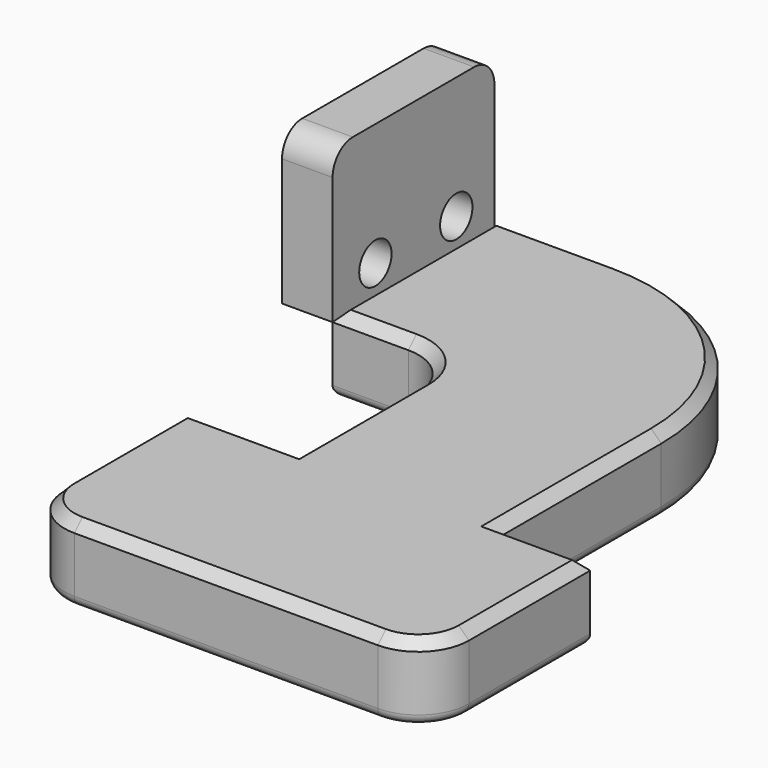
from build123d import *

# Parameters (mm, degrees)
F1_DEPTH = 7.5
F2_DEPTH = 2.5
F3_R     = 1
F4_SIZE  = 1
F5_R     = 2
F6_DEPTH = 5


# Not quite as in the source:
# - a feature names something its author has since deleted; it is built from what else it names


with BuildPart() as f1:
    # F0 (on Top) → F1 (new body)
    with BuildSketch(Plane.XY):
        with BuildLine():
            Line((-15.2574911714, 10), (-27.7574911714, 10))
            Line((-27.7574911714, 10), (-27.7574911714, -10))
            Line((-27.7574911714, -10), (-20.2574911714, -10))
            ThreePointArc((-20.2574911714, -10), (-16.7219572654, -11.4644660941), (-15.2574911714, -15))
            Line((-15.2574911714, -15), (-15.2574911714, -30.0000000031))
            Line((-15.2574911714, -30.0000000031), (4.7425088286, -30.0000000031))
            Line((4.7425088286, -30.0000000031), (4.7425088286, -10))
            ThreePointArc((4.7425088286, -10), (-1.1153555476, 4.1421356237), (-15.2574911714, 10))
        make_face()
        with BuildLine():
            Line((13.7208224833, -30.0000000031), (4.7425088286, -30.0000000031))
            Line((4.7425088286, -30.0000000031), (-15.2574911714, -30.0000000031))
            Line((-15.2574911714, -30.0000000031), (-26.2791775167, -30.0000000031))
            Line((-26.2791775167, -30.0000000031), (-26.2791775167, -45.0000000031))
            ThreePointArc((-26.2791775167, -45.0000000031), (-24.8147114226, -48.535533909), (-21.2791775167, -50.0000000031))
            Line((-21.2791775167, -50.0000000031), (8.7208224833, -50.0000000031))
            ThreePointArc((8.7208224833, -50.0000000031), (12.2563563892, -48.535533909), (13.7208224833, -45.0000000031))
            Line((13.7208224833, -45.0000000031), (13.7208224833, -30.0000000031))
        make_face()
    extrude(amount=-F1_DEPTH)

    # F0 (on Top) → F2 (join)
    with BuildSketch(Plane.XY):
        with BuildLine():
            Line((13.7208224833, -30.0000000031), (4.7425088286, -30.0000000031))
            Line((4.7425088286, -30.0000000031), (-15.2574911714, -30.0000000031))
            Line((-15.2574911714, -30.0000000031), (-26.2791775167, -30.0000000031))
            Line((-26.2791775167, -30.0000000031), (-26.2791775167, -45.0000000031))
            ThreePointArc((-26.2791775167, -45.0000000031), (-24.8147114226, -48.535533909), (-21.2791775167, -50.0000000031))
            Line((-21.2791775167, -50.0000000031), (8.7208224833, -50.0000000031))
            ThreePointArc((8.7208224833, -50.0000000031), (12.2563563892, -48.535533909), (13.7208224833, -45.0000000031))
            Line((13.7208224833, -45.0000000031), (13.7208224833, -30.0000000031))
        make_face()
    extrude(amount=-F2_DEPTH)

    # F3
    f3_edges = [f1.edges().sort_by_distance(p)[0] for p in [
        (-21.507491, 10, -7.5),
        (-27.757491, 0, -7.5),
        (-24.007491, -10, -7.5),
        (-16.721957, -11.464466, -7.5),
        (-15.257491, -22.5, -7.5),
        (-20.768334, -30, -7.5),
        (-26.279178, -37.5, -7.5),
        (-24.814711, -48.535534, -7.5),
        (-6.279178, -50, -7.5),
        (12.256356, -48.535534, -7.5),
        (13.720822, -37.5, -7.5),
        (9.231666, -30, -7.5),
        (4.742509, -20, -7.5),
        (-1.115356, 4.142136, -7.5),
    ]]
    fillet(f3_edges, radius=F3_R)

    # F4
    f4_edges = [f1.edges().sort_by_distance(p)[0] for p in [
        (-1.115356, 4.142136, 0),
        (-21.507491, 10, 0),
        (-27.757491, 0, 0),
        (-24.007491, -10, 0),
        (-16.721957, -11.464466, 0),
        (-15.257491, -22.5, 0),
        (-20.768334, -30, 0),
        (-26.279178, -37.5, 0),
        (-24.814711, -48.535534, 0),
        (-6.279178, -50, 0),
        (12.256356, -48.535534, 0),
        (13.720822, -37.5, 0),
        (9.231666, -30, 0),
        (4.742509, -20, 0),
    ]]
    chamfer(f4_edges, length=F4_SIZE)


with BuildPart() as f6:
    # F5 (on face) → F6 (new body)
    with BuildSketch(Plane(origin=(-27.7574911714, 0, 0), x_dir=(0, -1, 0), z_dir=(-1, 0, 0))):
        with BuildLine():
            Line((-10, 11.602570191), (-10, -1))
            Line((-10, -1), (10, -1))
            Line((10, -1), (10, 11.602570191))
            ThreePointArc((10, 11.602570191), (9.267766953, 13.370337144), (7.5, 14.102570191))
            Line((7.5, 14.102570191), (-7.5, 14.102570191))
            ThreePointArc((-7.5, 14.102570191), (-9.267766953, 13.370337144), (-10, 11.602570191))
        make_face()
        with BuildLine():
            ThreePointArc((-3.2897860792, 2), (-7.2845475439, 1.8553393662), (-3.3107127782, 2.2885634578))
            ThreePointArc((-3.3107127782, 2.2885634578), (-3.2950246145, 2.1446606338), (-3.2897860792, 2))
        make_face(mode=Mode.SUBTRACT)
        with Locations((4.7102139208, 2)):
            Circle(F5_R, mode=Mode.SUBTRACT)
    extrude(amount=F6_DEPTH)


solid = Compound([f1.part, f6.part])
